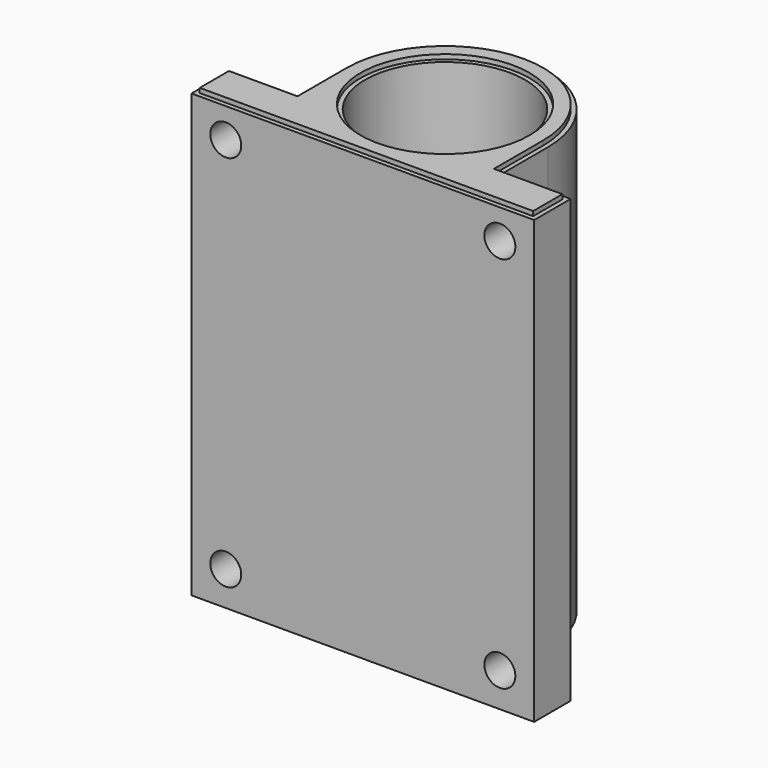
from build123d import *

# Parameters (mm, degrees)
F0_R     = 11.1125
F1_DEPTH = 62.0559846
F2_R     = 2.15265
F3_DEPTH = 6.35
F4_W     = 0.635
F4_H     = 0.635
F6_R     = 11.7475
F6_R_2   = 11.1125
F7_DEPTH = 0.635


# Not quite as in the source:
# - an extrude ends at something that could not be found from the text; its depth is read off the source's solid


with BuildPart() as f1:
    # F0 (on Top) → F1 (new body)
    with BuildSketch(Plane.XY):
        with BuildLine():
            ThreePointArc((14.2875, 0), (0, 14.2875), (-14.2875, 0))
            Line((-14.2875, 0), (-14.2875, -7.9375))
            Line((-14.2875, -7.9375), (-23.8125, -7.9375))
            Line((-23.8125, -7.9375), (-23.8125, -14.2875))
            Line((-23.8125, -14.2875), (23.8125, -14.2875))
            Line((23.8125, -14.2875), (23.8125, -7.9375))
            Line((23.8125, -7.9375), (14.2875, -7.9375))
            Line((14.2875, -7.9375), (14.2875, 0))
        make_face()
        Circle(F0_R, mode=Mode.SUBTRACT)
    extrude(amount=F1_DEPTH)

    # F2 (on face) → F3 (cut, through all)
    with BuildSketch(Plane.XZ.offset(14.2875)):
        with Locations((-19.05, 4.7625)):
            Circle(F2_R)
        with Locations((-19.05, 57.2934846)):
            Circle(F2_R)
        with Locations((19.05, 57.2934846)):
            Circle(F2_R)
        with Locations((19.05, 4.7625)):
            Circle(F2_R)
    extrude(amount=-F3_DEPTH, mode=Mode.SUBTRACT)

    # F5: sweep along a path in F5_path
    with BuildLine(Plane(origin=(23.8125, -14.2875, 62.0559846), x_dir=(0, -1, 0), z_dir=(0, 0, -1))) as f5_path:
        Line((0, 0), (0, 47.625))
        Line((0, 47.625), (-6.35, 47.625))
        Line((-6.35, 47.625), (-6.35, 38.1))
        Line((-6.35, 38.1), (-14.2875, 38.1))
        ThreePointArc((-14.2875, 38.1), (-28.575, 23.8125), (-14.2875, 9.525))
        Line((-14.2875, 9.525), (-6.35, 9.525))
        Line((-6.35, 9.525), (-6.35, 0))
        Line((-6.35, 0), (0, 0))
    # F4 (on face) → F5 (sweep, cut)
    with BuildSketch(Plane(origin=(-23.8125, 0, 0), x_dir=(0, -1, 0), z_dir=(-1, 0, 0))):
        with Locations((13.97, 61.7384846)):
            Rectangle(F4_W, F4_H)
    sweep(path=f5_path.line, transition=Transition.RIGHT, mode=Mode.SUBTRACT)

    # F6 (on face) → F7 (cut, through all)
    with BuildSketch(Plane.XY.offset(62.0559846)):
        Circle(F6_R)
        Circle(F6_R_2, mode=Mode.SUBTRACT)
    extrude(amount=-F7_DEPTH, mode=Mode.SUBTRACT)


solid = f1.part
